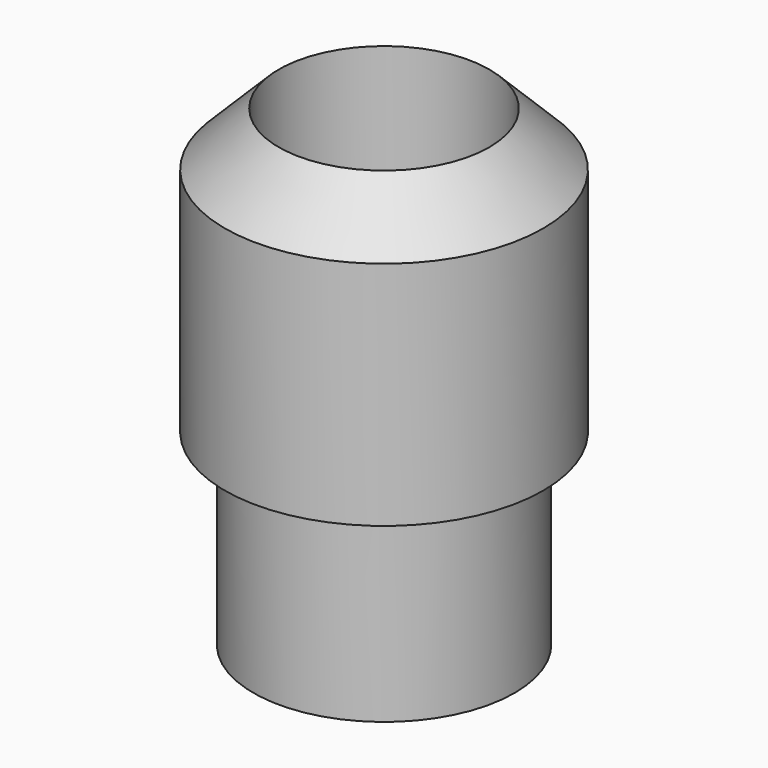
from build123d import *

# Parameters (mm, degrees)
F0_R     = 3.78
F1_DEPTH = 6.88
F2_R     = 3.1
F3_DEPTH = 4.45
F4_R     = 2.5
F5_DEPTH = 11.6


# Not quite as in the source:
# - a fillet or chamfer that OpenCascade refuses, or shapes differently, is made with other operations: its cross-section is extruded or revolved along the edge and cut away or added


with BuildPart() as f1:
    # F0 (on Top) → F1 (new body)
    with BuildSketch(Plane.XY):
        Circle(F0_R)
    extrude(amount=F1_DEPTH)

    # F2 (on face) → F3 (join)
    with BuildSketch(Plane(origin=(0, 0, 0), x_dir=(1, 0, 0), z_dir=(0, 0, -1))):
        Circle(F2_R)
    extrude(amount=F3_DEPTH)

    # F4 (on face) → F5 (cut)
    with BuildSketch(Plane.XY.offset(6.88)):
        Circle(F4_R)
    extrude(amount=-F5_DEPTH, mode=Mode.SUBTRACT)

    # F6: chamfer of 1.4 on 1 edges, made by hand

    # F6_s1 → F6_t2 (revolve, cut)
    with BuildSketch(Plane.XZ):
        Polygon((3.78, 5.48), (2.38, 6.88), (3.78, 6.88), align=None)
    revolve(axis=Axis((0, 0, 6.88), (0, 0, 1)), mode=Mode.SUBTRACT)


solid = f1.part
